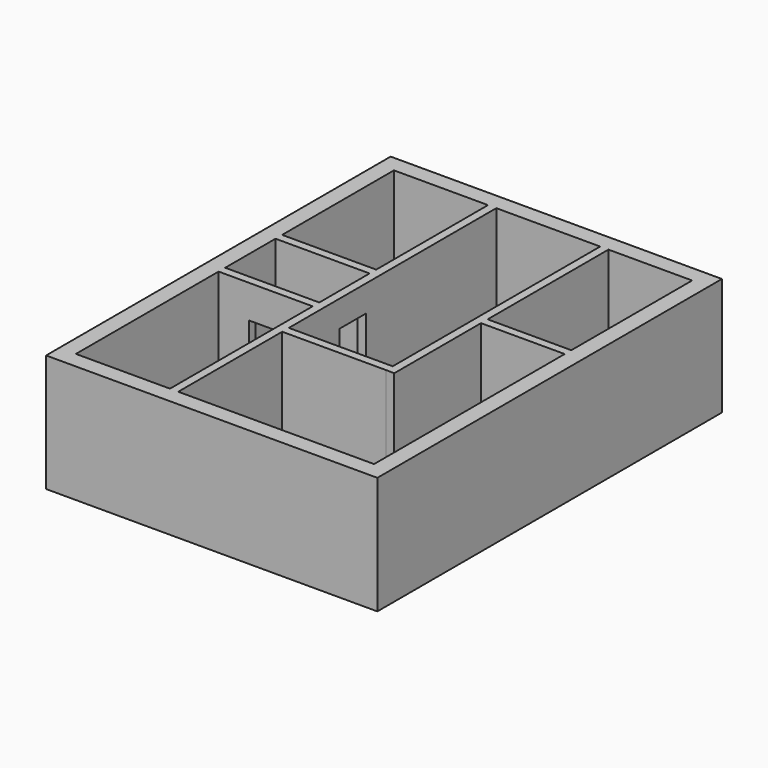
from build123d import *

# Parameters (mm, degrees)
F0_W      = 10000
F0_H      = 13000
F1_DEPTH  = 3550
F2_W      = 9000
F2_H      = 12000
F3_DEPTH  = 3300
F5_DEPTH  = 3300
F6_W      = 1000
F6_H      = 2300
F7_DEPTH  = 250
F8_W      = 1000
F8_H      = 2500
F9_DEPTH  = 250
F10_W     = 3135.6891602224
F10_H     = 2800
F11_DEPTH = 250


# Not quite as in the source:
# - a feature names something its author has since deleted; it is built from what else it names


with BuildPart() as f1:
    # F0 (on Top) → F1 (new body)
    with BuildSketch(Plane.XY):
        Rectangle(F0_W, F0_H)
    extrude(amount=F1_DEPTH)

    # F2 (on face) → F3 (cut)
    with BuildSketch(Plane.XY.offset(3550)):
        Rectangle(F2_W, F2_H)
    extrude(amount=-F3_DEPTH, mode=Mode.SUBTRACT)

    # F4 (on face) → F5 (join)
    with BuildSketch(Plane.XY.offset(250)):
        Polygon((-1660.4968309402, -366.6217029095), (-4500, -366.6217029095), (-4500, -616.6217029095), (-1660.4968309402, -616.6217029095), (-1660.4968309402, -6000), (-1410.4968309402, -6000), (-1410.4968309402, -2077.5351682588), (1725.1923292822, -2077.5351682588), (1975.1266148544, -2083.2669128011), (1975.1876689086, 1191.9026374817), (4500, 1191.9026374817), (4500, 1441.9026374817), (1975.1923292822, 1441.9026374817), (1975.1923292822, 6000), (1725.1923292822, 6000), (1725.1923292822, 1441.9026374817), (1725.1923292822, -1827.5351682588), (-1410.4968309402, -1827.5351682588), (-1410.4968309402, 6000), (-1660.4968309402, 6000), (-1660.4968309402, 1781.4515829086), (-4500, 1781.4515829086), (-4500, 1531.4515829086), (-1660.4968309402, 1531.4515829086), align=None)
    extrude(amount=F5_DEPTH)

    # F6 (on face) → F7 (cut)
    with BuildSketch(Plane.XZ.offset(616.6217029095)):
        with Locations((-3080.2484154701, 1400)):
            Rectangle(F6_W, F6_H)
    extrude(amount=-F7_DEPTH, mode=Mode.SUBTRACT)

    # F8 (on face) → F9 (cut, through all)
    with BuildSketch(Plane(origin=(-1660.4968309402, 0, 0), x_dir=(0, -1, 0), z_dir=(-1, 0, 0))):
        with Locations((-582.4149399996, 1500)):
            Rectangle(F8_W, F8_H)
    extrude(amount=-F9_DEPTH, mode=Mode.SUBTRACT)

    # F10 (on face) → F11 (cut, through all)
    with BuildSketch(Plane.XY.offset(250)):
        with Locations((157.347749171, 4600)):
            Rectangle(F10_W, F10_H)
    extrude(amount=-F11_DEPTH, mode=Mode.SUBTRACT)


solid = f1.part
